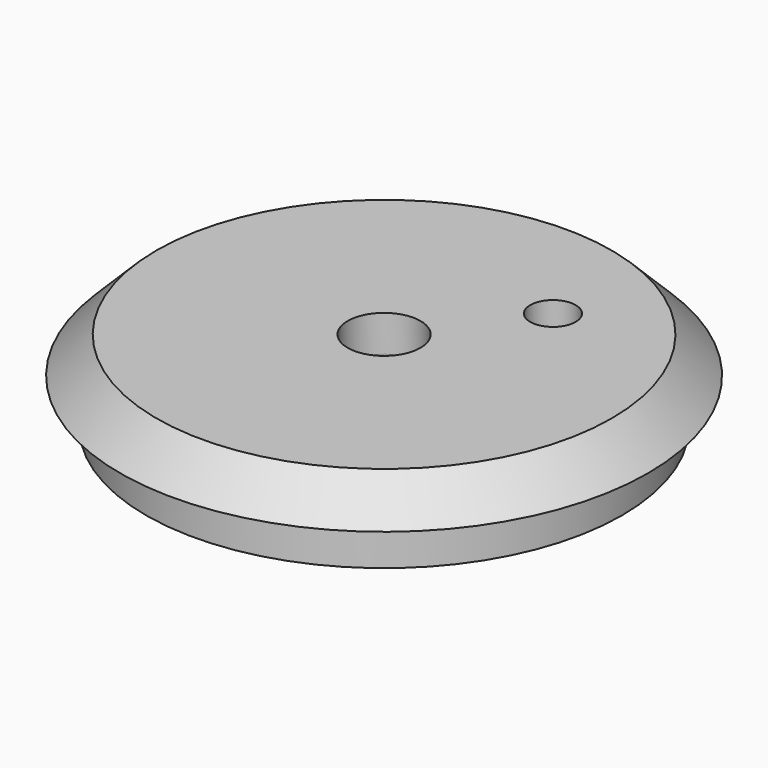
from build123d import *

# Parameters (mm, degrees)
F0_R          = 29
F1_DEPTH      = 4
F2_R          = 26.15
F3_DEPTH      = 5
F4_SIZE       = 3.99999
F5_R          = 4
F6_DEPTH      = 25
F6_DEPTH_BACK = 25
F7_R          = 2.5
F8_DEPTH      = 25
F8_DEPTH_BACK = 25


# Not quite as in the source:
# - a fillet or chamfer is up to 0.001 mm smaller than in the source, because OpenCascade refuses the exact size


with BuildPart() as f1:
    # F0 (on Top) → F1 (new body)
    with BuildSketch(Plane.XY):
        Circle(F0_R)
    extrude(amount=F1_DEPTH)

    # F2 (on Top) → F3 (join)
    with BuildSketch(Plane.XY):
        Circle(F2_R)
    extrude(amount=-F3_DEPTH)

    # F4 (size 4 in the source; OpenCascade refuses exactly that, so slightly less here)
    f4_edges = [f1.edges().sort_by_distance(p)[0] for p in [
        (-29, 0, 4),
    ]]
    chamfer(f4_edges, length=F4_SIZE)

    # F5 (on Top) → F6 (cut, two sides)
    with BuildSketch(Plane.XY) as f6_sk:
        Circle(F5_R)
    extrude(amount=F6_DEPTH, mode=Mode.SUBTRACT)
    extrude(f6_sk.sketch, amount=-F6_DEPTH_BACK, mode=Mode.SUBTRACT)

    # F7 (on Top) → F8 (cut, two sides)
    with BuildSketch(Plane.XY) as f8_sk:
        with Locations((8.8876162109, 12.0834712764)):
            Circle(F7_R)
    extrude(amount=F8_DEPTH, mode=Mode.SUBTRACT)
    extrude(f8_sk.sketch, amount=-F8_DEPTH_BACK, mode=Mode.SUBTRACT)


solid = f1.part
